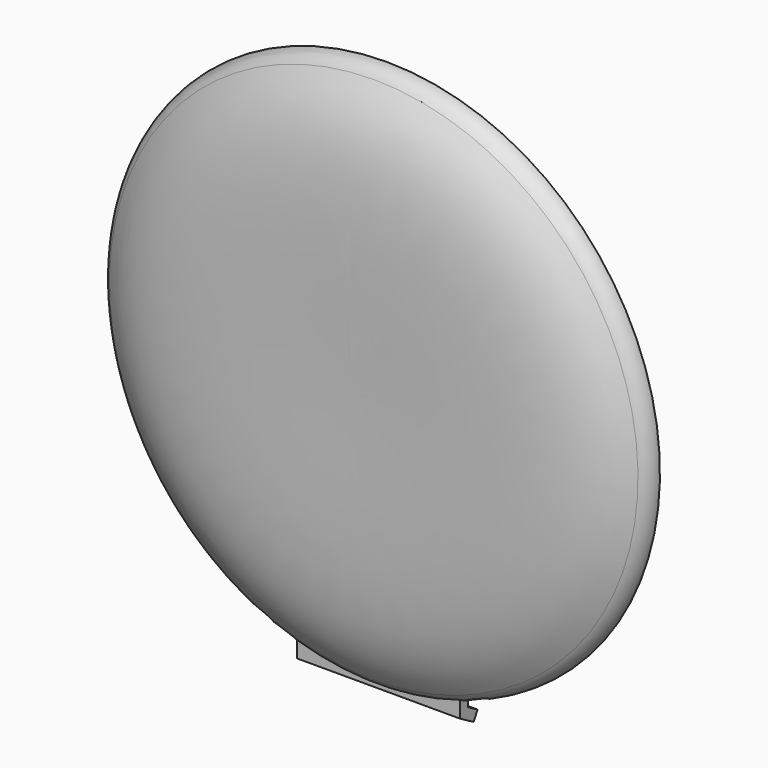
from build123d import *

# Parameters (mm, degrees)
F3_DEPTH = 1.27
F5_DEPTH = 20.32


# Not quite as in the source:
# - the dataset's text gives a spline's control points without its knots; the knots are read off the source's solid


with BuildPart() as f1:
    # F0 (on Right) → F1 (revolve)
    with BuildSketch(Plane.YZ):
        with BuildLine():
            Line((-5.5626, 0), (-3.175, 0))
            add(Edge.make_bspline(
                [(-3.175, 0), (-3.175, 10.541), (-4.0239762357, 25.9589322905), (-0.7943624519, 30.4792560231), (0, 31.75)],
                knots=[0, 0, 0, 0, 0.6813666235, 1, 1, 1, 1], degree=3))
            Line((0, 31.75), (0, 34.1376))
            ThreePointArc((0, 34.1376), (-1.1573462176, 33.8383446776), (-2.0245751497, 33.015594415))
            add(Edge.make_bspline(
                [(-5.5626, 0), (-5.5626, 1.9177725401), (-5.6012595175, 5.763256361), (-5.6850380944, 11.3740945743), (-5.7026900101, 16.6481342132), (-5.5838020802, 20.622627977), (-5.3557319657, 23.480741035), (-5.1437190397, 25.1246883423), (-4.9215103036, 26.3507670581), (-4.7229256392, 27.2307815663), (-4.4932831777, 28.052608441), (-4.1541081797, 29.0674517161), (-3.6792176979, 30.1931579589), (-2.8749355371, 31.7097687785), (-2.3121014901, 32.5556376731), (-2.0245751497, 33.015594415)],
                knots=[0, 0, 0, 0, 0.1249999999, 0.2499999998, 0.3749999996, 0.4999999995, 0.5624999995, 0.6249999994, 0.6562499994, 0.6874999993, 0.7187499993, 0.7499999993, 0.8124999992, 0.8749999991, 0.999999999, 0.999999999, 0.999999999, 0.999999999], degree=3))
        make_face()
    revolve(axis=Axis((0, -4.3688, 0), (0, 1, 0)))

    # F2 (on Front) → F3 (join)
    with BuildSketch(Plane.XZ):
        with BuildLine():
            Line((10.16, -34.2715069771), (10.16, -30.0805069771))
            ThreePointArc((10.16, -30.0805069771), (0, -31.75), (-10.16, -30.0805069771))
            Line((-10.16, -30.0805069771), (-10.16, -34.2715069771))
            Line((-10.16, -34.2715069771), (10.16, -34.2715069771))
        make_face()
    extrude(amount=F3_DEPTH)

    # F4 (on face) → F5 (join)
    with BuildSketch(Plane.YZ.offset(10.16)):
        Polygon((-0.635, -33.1716547143), (-1.27, -34.2715069771), (0.8637133898, -35.5034069771), (1.4987133898, -34.4035547143), align=None)
    extrude(amount=-F5_DEPTH)


solid = f1.part
